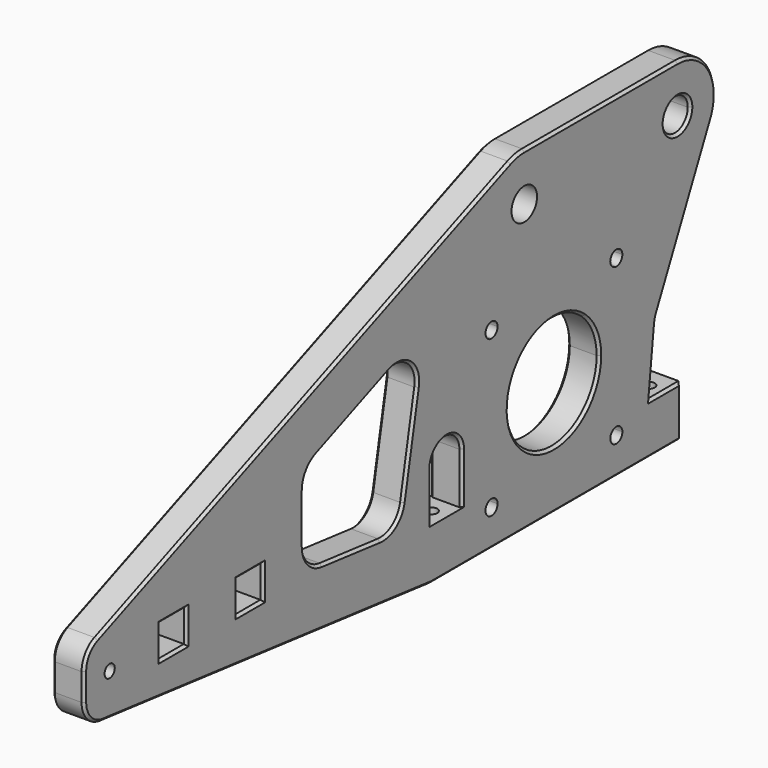
from build123d import *

# Parameters (mm, degrees)
F0_R     = 1.27
F0_R_2   = 3.175
F0_W     = 7.62
F0_H     = 10.16
F1_DEPTH = 6.35
F2_R     = 1.1938
F3_DEPTH = 10.16
F4_R     = 5.08
F5_SIZE  = 0.508


# Not quite as in the source:
# - a feature names something its author has since deleted; it is built from what else it names


with BuildPart() as f1:
    # F0 (on Right) → F1 (new body)
    with BuildSketch(Plane.YZ):
        with BuildLine():
            ThreePointArc((-44.8351920908, 6.7351920908), (-43.3633372108, 7.93869677), (-41.6817752313, 8.8259000217))
            Line((-41.6817752313, 8.8259000217), (-147.5800017288, -34.1503))
            Line((-147.5800017288, -34.1503), (-147.5800017288, -47.5107))
            Line((-147.5800017288, -47.5107), (-61.2200017288, -57.15))
            Line((-61.2200017288, -57.15), (-61.2200017288, -46.99))
            Line((-61.2200017288, -46.99), (-61.2200017288, -36.83))
            ThreePointArc((-61.2200017288, -36.83), (-57.4100017288, -33.02), (-53.6000017288, -36.83))
            Line((-53.6000017288, -36.83), (-53.6000017288, -2.0296175472))
            Line((-53.6000017288, -2.0296175472), (-44.8351920908, 6.7351920908))
        make_face()
        with Locations((-141.2300017288, -39.878)):
            Circle(F0_R, mode=Mode.SUBTRACT)
        Polygon((-122.1573017288, -36.6903), (-122.1573017288, -39.878), (-122.1573017288, -43.0657), (-128.5327017288, -43.0657), (-128.5327017288, -36.6903), align=None, mode=Mode.SUBTRACT)
        Polygon((-109.4827017288, -36.6903), (-103.1073017288, -36.6903), (-103.1073017288, -43.0657), (-109.4827017288, -43.0657), (-109.4827017288, -39.878), align=None, mode=Mode.SUBTRACT)
        Polygon((-92.9473017288, -24.3143284318), (-63.1243550698, -12.2114163884), (-69.2357549062, -44.7543205599), (-92.9473017288, -42.1076934955), align=None, mode=Mode.SUBTRACT)
        Polygon((-9.1300017288, -12.68), (-11.3668734516, -12.68), (-49.291932274, -12.68), (-52.3300017288, -36.875562325), (-52.3300017288, -55.88), (-9.963521833, -55.88), (-9.1300017288, -53.5610139018), align=None)
        with BuildLine():
            ThreePointArc((-16.7047434898, -18.6345126787), (-16.3269172867, -17.7587509619), (-15.4975041416, -17.287810351))
            ThreePointArc((-15.4975041416, -17.287810351), (-14.2563911214, -17.6021456009), (-13.7100017288, -18.76))
            ThreePointArc((-13.7100017288, -18.76), (-14.149341557, -19.8206601718), (-15.2100017288, -20.26))
            Line((-15.2100017288, -20.26), (-15.2100017288, -48.3))
            ThreePointArc((-15.2100017288, -48.3), (-14.149341557, -48.7393398282), (-13.7100017288, -49.8))
            ThreePointArc((-13.7100017288, -49.8), (-15.2100017288, -51.3), (-16.7100017288, -49.8))
            Line((-16.7100017288, -49.8), (-44.7500017288, -49.8))
            ThreePointArc((-44.7500017288, -49.8), (-47.3106619005, -50.8606601718), (-46.2500017288, -48.3))
            Line((-46.2500017288, -48.3), (-46.2500017288, -20.26))
            ThreePointArc((-46.2500017288, -20.26), (-47.3106619005, -17.6993398282), (-44.7500017288, -18.76))
            Line((-44.7500017288, -18.76), (-16.8172354852, -18.76))
            Line((-16.8172354852, -18.76), (-16.7047434898, -18.6345126787))
        make_face(mode=Mode.SUBTRACT)
        with BuildLine():
            Line((-16.7100017288, -18.76), (-16.8172354852, -18.76))
            Line((-16.8172354852, -18.76), (-44.7500017288, -18.76))
            ThreePointArc((-44.7500017288, -18.76), (-45.189341557, -19.8206601718), (-46.2500017288, -20.26))
            Line((-46.2500017288, -20.26), (-46.2500017288, -48.3))
            ThreePointArc((-46.2500017288, -48.3), (-45.189341557, -48.7393398282), (-44.7500017288, -49.8))
            Line((-44.7500017288, -49.8), (-16.7100017288, -49.8))
            ThreePointArc((-16.7100017288, -49.8), (-16.2706619005, -48.7393398282), (-15.2100017288, -48.3))
            Line((-15.2100017288, -48.3), (-15.2100017288, -20.26))
            ThreePointArc((-15.2100017288, -20.26), (-16.2706619005, -19.8206601718), (-16.7100017288, -18.76))
        make_face()
        with BuildLine():
            ThreePointArc((-19.4800017288, -34.28), (-41.0023648355, -38.8670531067), (-23.2206339428, -25.9031333152))
            ThreePointArc((-23.2206339428, -25.9031333152), (-20.457638622, -29.6929468933), (-19.4800017288, -34.28))
        make_face(mode=Mode.SUBTRACT)
        with BuildLine():
            Line((-11.3668734516, -12.68), (-6.3579313922, -7.0924137931))
            ThreePointArc((-6.3579313922, -7.0924137931), (-8.8960908937, 3.4037026619), (0, 9.525))
            Line((0, 9.525), (-38.1, 9.525))
            ThreePointArc((-38.1, 9.525), (-31.3648079092, 6.7351920908), (-28.575, 0))
            ThreePointArc((-28.575, 0), (-38.6944942594, -9.5064294862), (-47.5507903571, 1.1866703952))
            Line((-47.5507903571, 1.1866703952), (-49.291932274, -12.68))
            Line((-49.291932274, -12.68), (-11.3668734516, -12.68))
        make_face()
        with BuildLine():
            ThreePointArc((8.6073212119, -4.0791722879), (1.8801182762, -9.3376003485), (-6.3579313922, -7.0924137931))
            Line((-6.3579313922, -7.0924137931), (-11.3668734516, -12.68))
            Line((-11.3668734516, -12.68), (-9.1300017288, -12.68))
            Line((-9.1300017288, -12.68), (-9.1300017288, -53.5610139018))
            Line((-9.1300017288, -53.5610139018), (-6.7681625627, -46.99))
            Line((-6.7681625627, -46.99), (-5.248416905, -33.3156889593))
            Line((-5.248416905, -33.3156889593), (8.6073212119, -4.0791722879))
        make_face()
        with BuildLine():
            ThreePointArc((-28.575, 0), (-31.3648079092, 6.7351920908), (-38.1, 9.525))
            ThreePointArc((-38.1, 9.525), (-39.9246817933, 9.3485914101), (-41.6817752313, 8.8259000217))
            ThreePointArc((-41.6817752313, 8.8259000217), (-43.3633372108, 7.93869677), (-44.8351920908, 6.7351920908))
            ThreePointArc((-44.8351920908, 6.7351920908), (-46.6552925258, 4.1871941438), (-47.5507903571, 1.1866703952))
            ThreePointArc((-47.5507903571, 1.1866703952), (-38.6944942594, -9.5064294862), (-28.575, 0))
        make_face()
        with Locations((-38.1, 0)):
            Circle(F0_R_2, mode=Mode.SUBTRACT)
        with BuildLine():
            ThreePointArc((0, 9.525), (-8.8960908937, 3.4037026619), (-6.3579313922, -7.0924137931))
            ThreePointArc((-6.3579313922, -7.0924137931), (1.8801182762, -9.3376003485), (8.6073212119, -4.0791722879))
            ThreePointArc((8.6073212119, -4.0791722879), (8.7958988014, -3.6548309503), (8.9635712281, -3.2218031967))
            ThreePointArc((8.9635712281, -3.2218031967), (9.3835931537, -1.6351772155), (9.525, 0))
            ThreePointArc((9.525, 0), (6.7351920908, 6.7351920908), (0, 9.525))
        make_face()
        with BuildLine():
            ThreePointArc((-2.1277877059, -2.3735944828), (-1.2997465945, 2.9106855), (3.1877, 0))
            ThreePointArc((3.1877, 0), (1.2997465945, -2.9106855), (-2.1277877059, -2.3735944828))
        make_face(mode=Mode.SUBTRACT)
        with BuildLine():
            Line((-52.3300017288, -12.68), (-49.291932274, -12.68))
            Line((-49.291932274, -12.68), (-47.5507903571, 1.1866703952))
            ThreePointArc((-47.5507903571, 1.1866703952), (-46.6552925258, 4.1871941438), (-44.8351920908, 6.7351920908))
            Line((-44.8351920908, 6.7351920908), (-53.6000017288, -2.0296175472))
            Line((-53.6000017288, -2.0296175472), (-53.6000017288, -36.83))
            Line((-53.6000017288, -36.83), (-53.6000017288, -46.99))
            Line((-53.6000017288, -46.99), (-52.3300017288, -36.875562325))
            Line((-52.3300017288, -36.875562325), (-52.3300017288, -12.68))
        make_face()
        Polygon((0.8518374373, -46.99), (-6.7681625627, -46.99), (-9.1300017288, -53.5610139018), (-9.1300017288, -55.88), (-9.963521833, -55.88), (-10.4200017288, -57.15), (0.8518374373, -57.15), align=None)
        with Locations((-57.4100017288, -52.07)):
            Rectangle(F0_W, F0_H)
        Polygon((-52.3300017288, -55.88), (-52.3300017288, -36.875562325), (-53.6000017288, -46.99), (-53.6000017288, -57.15), (-10.4200017288, -57.15), (-9.963521833, -55.88), align=None)
        Polygon((-52.3300017288, -36.875562325), (-49.291932274, -12.68), (-52.3300017288, -12.68), align=None)
        Polygon((-9.1300017288, -55.88), (-9.1300017288, -53.5610139018), (-9.963521833, -55.88), align=None)
    extrude(amount=-F1_DEPTH)

    # F2 (on face) → F3 (cut, through all)
    with BuildSketch(Plane(origin=(0, 0, -57.15), x_dir=(1, 0, 0), z_dir=(0, 0, -1))):
        with Locations((-3.175, 57.2830017288)):
            Circle(F2_R)
        with Locations((-3.175, 3.1810017288)):
            Circle(F2_R)
    extrude(amount=-F3_DEPTH, mode=Mode.SUBTRACT)

    # F4
    f4_edges = [f1.edges().sort_by_distance(p)[0] for p in [
        (-3.175, -147.580002, -34.1503),
        (-3.175, -147.580002, -47.5107),
        (-3.175, -69.235755, -44.754321),
        (-3.175, -92.947302, -42.107693),
        (-3.175, -92.947302, -24.314328),
        (-3.175, -63.124355, -12.211416),
        (-3.175, -5.248417, -33.315689),
    ]]
    fillet(f4_edges, radius=F4_R)

    # F5
    f5_edges = [f1.edges().sort_by_distance(p)[0] for p in [
        (0, -93.046029, -12.019023),
        (0, -30.184082, -57.15),
        (0, 0.851837, -52.07),
        (-6.35, 0.851837, -52.07),
        (-6.35, -30.184082, -57.15),
        (-6.35, -102.141761, -52.58241),
        (0, -81.17628, -43.421547),
        (-6.35, -106.295002, -36.6903),
        (-6.35, -103.107302, -39.878),
        (-6.35, -106.295002, -43.0657),
        (-6.35, -109.482702, -39.878),
        (-6.35, -122.157302, -39.878),
        (-6.35, -125.345002, -43.0657),
        (-6.35, -128.532702, -39.878),
        (-6.35, -125.345002, -36.6903),
        (0, -125.345002, -36.6903),
        (0, -128.532702, -39.878),
        (0, -125.345002, -43.0657),
        (0, -122.157302, -39.878),
        (0, -106.295002, -43.0657),
        (0, -109.482702, -39.878),
        (0, -106.295002, -36.6903),
        (0, -103.107302, -39.878),
        (0, -61.220002, -41.91),
        (-6.35, -61.220002, -41.91),
        (-3.175, -23.220634, -25.903133),
        (0, -38.23937, -42.656867),
        (-6.35, -38.23937, -42.656867),
        (-6.35, -2.958163, -46.99),
        (0, -2.958163, -46.99),
        (-6.35, -81.17628, -43.421547),
        (-3.175, -2.127788, -2.373594),
        (0, 2.127788, 2.373594),
        (-6.35, 2.127788, 2.373594),
        (0, 1.861634, -18.313014),
        (-6.35, 1.861634, -18.313014),
        (0, -146.713707, -34.73365),
        (0, -39.924682, 9.348591),
        (0, -147.580002, -40.268632),
        (0, -19.05, 9.525),
        (0, -146.286099, -46.353185),
        (0, 8.049216, 5.092716),
        (0, -102.141761, -52.58241),
        (0, -5.180353, -33.335013),
        (0, -6.055279, -40.575643),
        (0, -57.410002, -33.02),
        (0, -53.600002, -41.91),
        (0, -66.60343, -30.737318),
        (0, -66.618314, -16.484199),
        (0, -70.336694, -43.266355),
        (0, -80.760974, -19.368806),
        (0, -92.081007, -24.897678),
        (0, -91.653399, -40.950178),
        (0, -92.947302, -32.649143),
        (-6.35, -5.180353, -33.335013),
        (-6.35, 8.049216, 5.092716),
        (-6.35, -93.046029, -12.019023),
        (-6.35, -146.713707, -34.73365),
        (-6.35, -39.924682, 9.348591),
        (-6.35, -147.580002, -40.268632),
        (-6.35, -19.05, 9.525),
        (-6.35, -146.286099, -46.353185),
        (-6.35, -6.055279, -40.575643),
        (-6.35, -57.410002, -33.02),
        (-6.35, -53.600002, -41.91),
        (-6.35, -66.60343, -30.737318),
        (-6.35, -66.618314, -16.484199),
        (-6.35, -70.336694, -43.266355),
        (-6.35, -80.760974, -19.368806),
        (-6.35, -92.081007, -24.897678),
        (-6.35, -91.653399, -40.950178),
        (-6.35, -92.947302, -32.649143),
    ]]
    chamfer(f5_edges, length=F5_SIZE)


solid = f1.part
